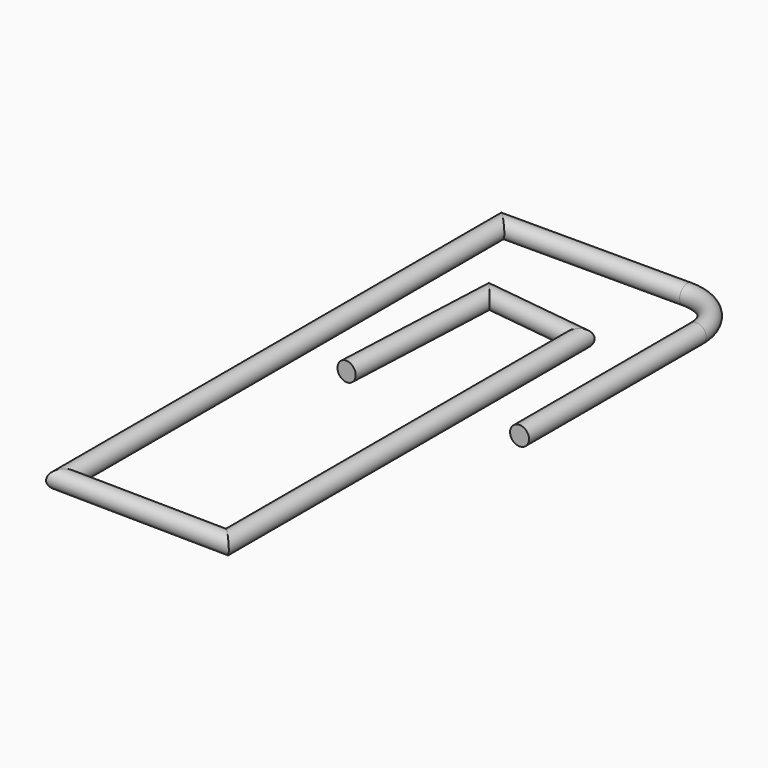
from build123d import *

# Parameters (mm, degrees)
F0_R = 1.27


with BuildPart() as f2:
    # F2: sweep along a path in F1
    with BuildLine(Plane.XY) as f2_path:
        Line((0, 0), (0, 29.7363953829))
        ThreePointArc((0, 29.7363953829), (-1.8598719395, 34.2265234434), (-6.35, 36.0863953829))
        Line((-6.35, 36.0863953829), (-31.1682708561, 36.0863953829))
        Line((-31.1682708561, 36.0863953829), (-31.1682708561, -37.6992039382))
        Line((-31.1682708561, -37.6992039382), (-8.8609969243, -38.042396307))
        Line((-8.8609969243, -38.042396307), (-8.8609969243, 20.9860876203))
        Line((-8.8609969243, 20.9860876203), (-22.2453605384, 22.7020308375))
        Line((-22.2453605384, 22.7020308375), (-23.2749264687, 0.0515673637))
    # F0 (on Front) → F2 (sweep)
    with BuildSketch(Plane.XZ):
        Circle(F0_R)
    sweep(path=f2_path.line, transition=Transition.RIGHT)


solid = f2.part
